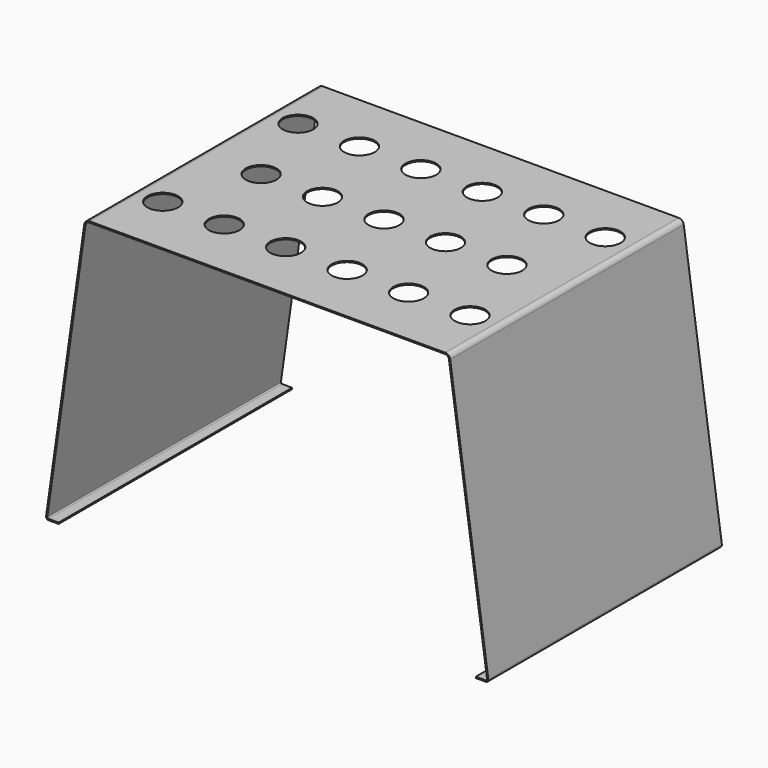
from build123d import *

# Parameters (mm, degrees)
F1_DEPTH = 723.9
F2_R     = 38.1
F3_DEPTH = 25.4


# Not quite as in the source:
# - ends of sketch curves that miss each other by under 0.0002 mm in the source are joined


with BuildPart() as f1:
    # F0 (on Front) → F1 (new body)
    with BuildSketch(Plane.XZ):
        with BuildLine():
            ThreePointArc((-8215.9952266, 774.938506), (-8224.3216631827, 771.8281073386), (-8228.56958997, 764.0204672337))
            Line((-8228.56958997, 764.0204672337), (-8323.1839632, 96.3794872))
            ThreePointArc((-8323.1839632, 96.3794872), (-8321.6915780693, 91.3252877086), (-8316.8967774, 89.138506))
            Line((-8316.8967774, 89.138506), (-8292.1428772, 89.138506))
            Line((-8292.1428772, 89.138506), (-8292.1428772, 92.313506))
            Line((-8292.1428772, 92.313506), (-8317.8109488, 92.313506))
            ThreePointArc((-8317.8109488, 92.313506), (-8319.6089965519, 93.1335462625), (-8320.1686430016, 95.0288661831))
            Line((-8320.1686430016, 95.0288661831), (-8225.4259926, 763.5749778))
            ThreePointArc((-8225.4259926, 763.5749778), (-8222.2400533643, 769.4307075881), (-8215.9952266, 771.763506))
            Line((-8215.9952266, 771.763506), (-7333.739841, 771.763506))
            ThreePointArc((-7333.739841, 771.763506), (-7327.4950142357, 769.4307075881), (-7324.3090687225, 763.5749786896))
            Line((-7324.3090687225, 763.5749786896), (-7229.6946846, 95.9339966))
            ThreePointArc((-7229.6946846, 95.9339966), (-7230.4408638812, 93.4068975271), (-7232.8382648, 92.313506))
            Line((-7232.8382648, 92.313506), (-7257.592165, 92.313506))
            Line((-7257.592165, 92.313506), (-7257.592165, 89.138506))
            Line((-7257.592165, 89.138506), (-7232.8382648, 89.138506))
            ThreePointArc((-7232.8382648, 89.138506), (-7228.0434641307, 91.3252877086), (-7226.551083115, 96.3794866168))
            Line((-7226.551083115, 96.3794866168), (-7321.1654694, 764.0204684))
            ThreePointArc((-7321.1654694, 764.0204684), (-7325.4134044173, 771.8281073386), (-7333.739841, 774.938506))
            Line((-7333.739841, 774.938506), (-8215.9952266, 774.938506))
        make_face()
    extrude(amount=F1_DEPTH)

    # F2 (on face) → F3 (cut)
    with BuildSketch(Plane.XY.offset(774.938506)):
        with Locations((-8155.8675338, -152.4)):
            Circle(F2_R)
        with Locations((-8003.4675338, -152.4)):
            Circle(F2_R)
        with Locations((-7851.0675338, -152.4)):
            Circle(F2_R)
        with Locations((-7698.6675338, -152.4)):
            Circle(F2_R)
        with Locations((-7546.2675338, -152.4)):
            Circle(F2_R)
        with Locations((-7393.8675338, -152.4)):
            Circle(F2_R)
        with Locations((-8079.6675338, -361.95)):
            Circle(F2_R)
        with Locations((-7927.2675338, -361.95)):
            Circle(F2_R)
        with Locations((-7774.8675338, -361.95)):
            Circle(F2_R)
        with Locations((-7622.4675338, -361.95)):
            Circle(F2_R)
        with Locations((-7470.0675338, -361.95)):
            Circle(F2_R)
        with Locations((-8155.8675338, -571.5)):
            Circle(F2_R)
        with Locations((-8003.4675338, -571.5)):
            Circle(F2_R)
        with Locations((-7851.0675338, -571.5)):
            Circle(F2_R)
        with Locations((-7698.6675338, -571.5)):
            Circle(F2_R)
        with Locations((-7546.2675338, -571.5)):
            Circle(F2_R)
        with Locations((-7393.8675338, -571.5)):
            Circle(F2_R)
    extrude(amount=-F3_DEPTH, mode=Mode.SUBTRACT)


solid = f1.part
